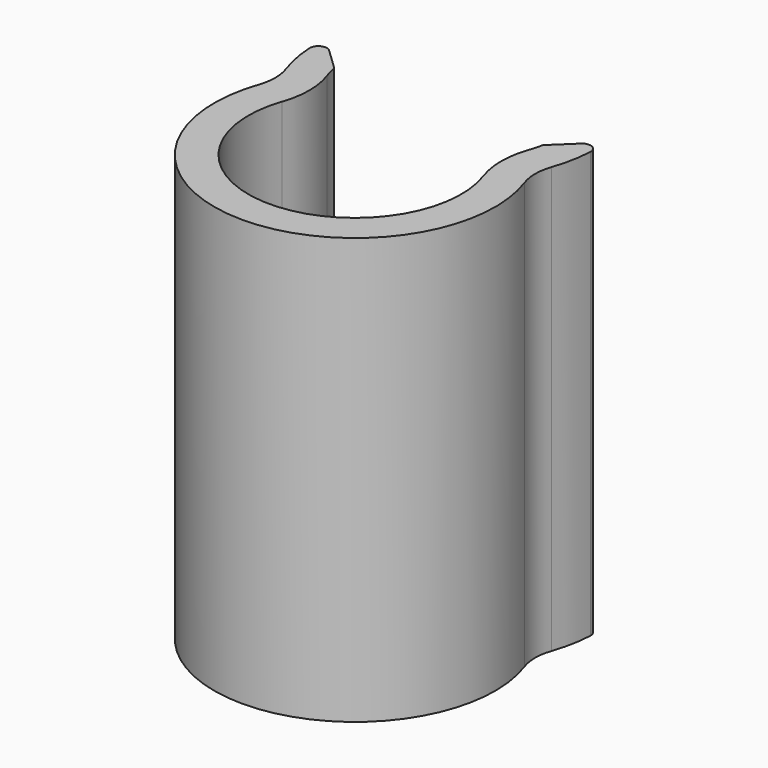
from build123d import *

# Parameters (mm, degrees)
F1_DEPTH = 10


# Not quite as in the source:
# - a feature names something its author has since deleted; it is built from what else it names


with BuildPart() as f1:
    # F0 (on Top) → F1 (new body)
    with BuildSketch(Plane.XY):
        with BuildLine():
            ThreePointArc((2.3611111111, 0.8216777477), (0, -2.5), (-2.3611111111, 0.8216777477))
            ThreePointArc((-2.3611111111, 0.8216777477), (-2.25, 1.4790199458), (-2.3611111111, 2.1363621439))
            ThreePointArc((-2.3611111111, 2.1363621439), (-2.4106719576, 2.2957252286), (-2.4494897428, 2.4580398915))
            Line((-2.4494897428, 2.4580398915), (-2.9577320216, 2.9439046938))
            ThreePointArc((-2.9577320216, 2.9439046938), (-3.1792292558, 2.9811663012), (-3.2956726945, 2.7890976215))
            ThreePointArc((-3.2956726945, 2.7890976215), (-3.2386938705, 2.3249032452), (-3.1166666667, 1.8734252646))
            ThreePointArc((-3.1166666667, 1.8734252646), (-3.05, 1.4790199458), (-3.1166666667, 1.0846146269))
            ThreePointArc((-3.1166666667, 1.0846146269), (0, -3.3), (3.1166666667, 1.0846146269))
            ThreePointArc((3.1166666667, 1.0846146269), (3.05, 1.4790199458), (3.1166666667, 1.8734252646))
            ThreePointArc((3.1166666667, 1.8734252646), (3.2386938705, 2.3249032452), (3.2956726945, 2.7890976215))
            ThreePointArc((3.2956726945, 2.7890976215), (3.1792292558, 2.9811663012), (2.9577320216, 2.9439046938))
            Line((2.9577320216, 2.9439046938), (2.4494897428, 2.4580398915))
            ThreePointArc((2.4494897428, 2.4580398915), (2.4106719576, 2.2957252286), (2.3611111111, 2.1363621439))
            ThreePointArc((2.3611111111, 2.1363621439), (2.25, 1.4790199458), (2.3611111111, 0.8216777477))
        make_face()
    extrude(amount=F1_DEPTH)


solid = f1.part
